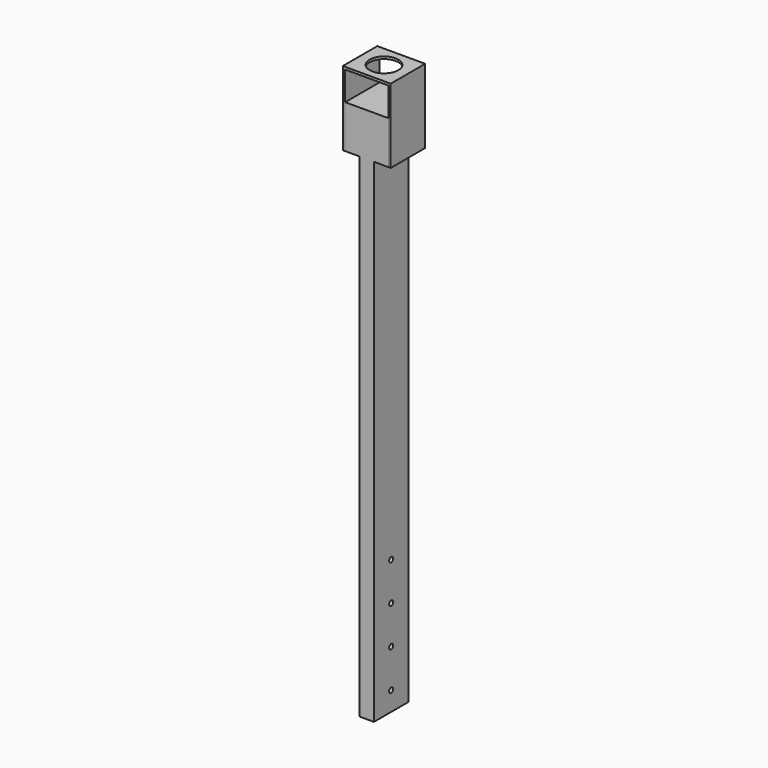
from build123d import *

# Parameters (mm, degrees)
F0_W      = 19.05
F0_H      = 57.15
F1_DEPTH  = 711.2
F2_W      = 57.15
F2_H      = 57.15
F3_DEPTH  = 19.05
F4_W      = 57.15
F4_H      = 57.15
F5_DEPTH  = 19.05
F7_W      = 57.15
F7_H      = 57.15
F7_W_2    = 3.175
F8_DEPTH  = 3.175
F9_W      = 3.175
F9_H      = 57.15
F10_DEPTH = 95.25
F11_R     = 19.05
F12_DEPTH = 3.175
F13_R     = 3.302
F14_DEPTH = 19.05


with BuildPart() as f1:
    # F0 (on Top) → F1 (new body)
    with BuildSketch(Plane.XY):
        with Locations((9.525, 28.575)):
            Rectangle(F0_W, F0_H)
    extrude(amount=F1_DEPTH)

    # F2 (on face) → F3 (join)
    with BuildSketch(Plane(origin=(0, 0, 0), x_dir=(0, -1, 0), z_dir=(-1, 0, 0))):
        with Locations((-28.575, 682.625)):
            Rectangle(F2_W, F2_H)
    extrude(amount=F3_DEPTH)

    # F4 (on face) → F5 (join)
    with BuildSketch(Plane.YZ.offset(19.05)):
        with Locations((28.575, 682.625)):
            Rectangle(F4_W, F4_H)
    extrude(amount=F5_DEPTH)

    # F13 (on face) → F14 (cut, through all)
    with BuildSketch(Plane(origin=(0, 0, 0), x_dir=(0, -1, 0), z_dir=(-1, 0, 0))):
        with Locations((-28.575, 25.4)):
            Circle(F13_R)
        with Locations((-28.575, 76.2)):
            Circle(F13_R)
        with Locations((-28.575, 127)):
            Circle(F13_R)
        with Locations((-28.575, 177.8)):
            Circle(F13_R)
    extrude(amount=-F14_DEPTH, mode=Mode.SUBTRACT)


with BuildPart() as f8:
    # F7 (on offset) → F8 (new body)
    with BuildSketch(Plane.XY.offset(749.3)):
        with Locations((9.525, 28.575)):
            Rectangle(F7_W, F7_H)
        with Locations((39.6875, 28.575)):
            Rectangle(F7_W_2, F7_H)
        with Locations((-20.6375, 28.575)):
            Rectangle(F7_W_2, F7_H)
    extrude(amount=F8_DEPTH)

    # F9 (on face) → F10 (join, through all)
    with BuildSketch(Plane(origin=(0, 0, 749.3), x_dir=(1, 0, 0), z_dir=(0, 0, -1))):
        with Locations((-20.6375, -28.575)):
            Rectangle(F9_W, F9_H)
        with Locations((39.6875, -28.575)):
            Rectangle(F9_W, F9_H)
    extrude(amount=F10_DEPTH)

    # F11 (on face) → F12 (cut, through all)
    with BuildSketch(Plane.XY.offset(752.475)):
        with Locations((9.525, 28.575)):
            Circle(F11_R)
    extrude(amount=-F12_DEPTH, mode=Mode.SUBTRACT)


solid = Compound([f1.part, f8.part])
